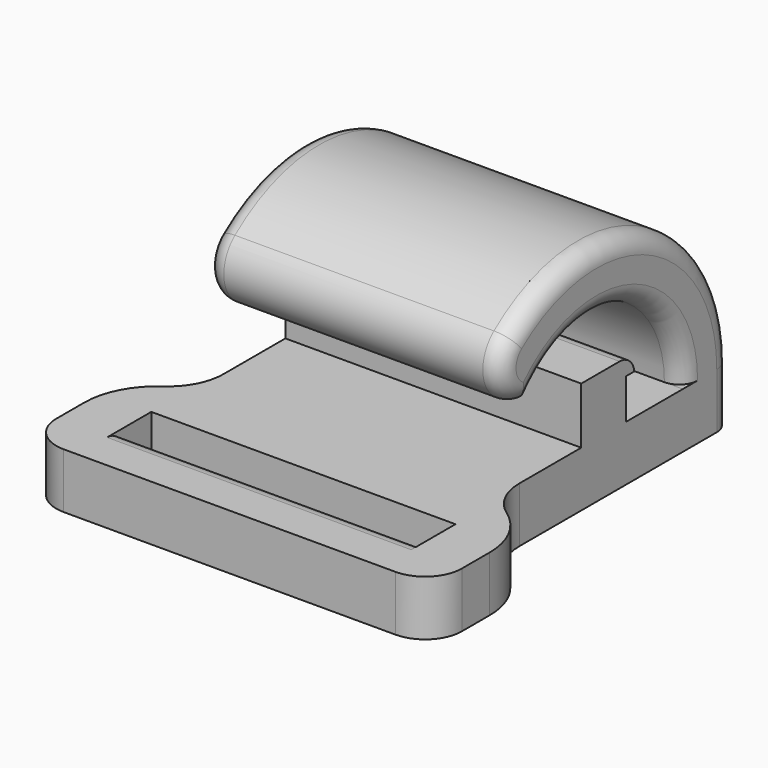
from build123d import *

# Parameters (mm, degrees)
F3_DEPTH       = 16.05
F4_W           = 5.4241176695
F4_H           = 3.5927895224
F5_DEPTH       = 25
F5_DEPTH_BACK  = 25
F6_T1_DEPTH    = 38.39224199
F8_DEPTH       = 8.025
F8_DEPTH_BACK  = 8.025
F9_T1_DEPTH    = 21.0152154422
F11_W          = 7.7522003338
F11_H          = 3
F12_DEPTH      = 11
F12_DEPTH_BACK = 11
F13_W          = 16.5
F13_H          = 2
F14_DEPTH      = 25
F15_R          = 1
F16_T1_DEPTH   = 22.3322108151
F17_T3_ANGLE   = 128.6137584612
F17_T6_ANGLE   = 128.6137584612
F17_T9_ANGLE   = 166.6195765903
F17_T12_ANGLE  = 166.6195765903
F17_T15_ANGLE  = 208.6372867238
F17_T18_ANGLE  = 208.6372867238
F17_T21_DEPTH  = 5.5
F17_T24_DEPTH  = 5.5
F18_R          = 2
F19_R          = 3


# Not quite as in the source:
# - a fillet or chamfer that OpenCascade refuses, or shapes differently, is made with other operations: its cross-section is extruded or revolved along the edge and cut away or added


with BuildPart() as f3:
    # F2 (on line) → F3 (new body)
    with BuildSketch(Plane.YZ.offset(-8.025)):
        with BuildLine():
            Line((30.8775485963, 0), (34.1775485963, 0))
            ThreePointArc((34.1775485963, 0), (25.0275485963, 9.15), (15.8775485963, 0))
            Line((15.8775485963, 0), (19.1775485963, 0))
            ThreePointArc((19.1775485963, 0), (25.0275485963, 5.85), (30.8775485963, 0))
        make_face()
    extrude(amount=F3_DEPTH)

    # F4 (on Right) → F5 (cut, two sides)
    with BuildSketch(Plane.YZ) as f5_sk:
        with Locations((17.9089335725, 1.7963947612)):
            Rectangle(F4_W, F4_H)
    extrude(amount=-F5_DEPTH, mode=Mode.SUBTRACT)
    extrude(f5_sk.sketch, amount=F5_DEPTH_BACK, mode=Mode.SUBTRACT)

    # F6: fillet of radius 2 on 1 edges, made by hand

    # F6_s2 → F6_t1 (cut)
    with BuildSketch(Plane.YZ.offset(-19.196120995)):
        with BuildLine():
            ThreePointArc((19.3173332992, 7.1495413322), (18.6537711345, 4.9990791235), (20.4108004498, 3.5927895224))
            Line((20.4108004498, 3.5927895224), (16.6124215356, 3.5927895224))
            ThreePointArc((16.6124215356, 3.5927895224), (17.7444211746, 5.5388225246), (19.3173332992, 7.1495413322))
        make_face()
    extrude(amount=F6_T1_DEPTH, mode=Mode.SUBTRACT)

    # F7 (on Right) → F8 (join, two sides)
    with BuildSketch(Plane.YZ) as f8_sk:
        Polygon((34.1775485963, 0), (27.0130820572, 0), (23.9856019616, 0), (10.1775485963, 0), (10.1775485963, -3), (34.1775485963, -3), align=None)
        Polygon((23.9856019616, 0), (27.0130820572, 0), (27.0130820572, 2.18), (27.5856019616, 2.18), (27.5856019616, 3.0622484628), (23.9856019616, 3.0622484628), (23.9856019616, 2.18), align=None)
    extrude(amount=F8_DEPTH)
    extrude(f8_sk.sketch, amount=-F8_DEPTH_BACK)

    # F9: fillet of radius 1 on 1 edges, made by hand

    # F9_s2 → F9_t1 (cut)
    with BuildSketch(Plane.YZ.offset(-10.5076077211)):
        with BuildLine():
            ThreePointArc((27.5856019616, 2.18), (27.2567307119, 2.8098284041), (26.5925588732, 3.0622484628))
            Line((26.5925588732, 3.0622484628), (27.5856019616, 3.0622484628))
            Line((27.5856019616, 3.0622484628), (27.5856019616, 2.18))
        make_face()
    extrude(amount=F9_T1_DEPTH, mode=Mode.SUBTRACT)

    # F10: union 

    # F11 (on Right) → F12 (join, two sides)
    with BuildSketch(Plane.YZ) as f12_sk:
        with Locations((14.0536487631, -1.5)):
            Rectangle(F11_W, F11_H)
    extrude(amount=F12_DEPTH)
    extrude(f12_sk.sketch, amount=-F12_DEPTH_BACK)

    # F13 (on Top) → F14 (cut)
    with BuildSketch(Plane.XY):
        with Locations((0, 14.1775485963)):
            Rectangle(F13_W, F13_H)
    extrude(amount=-F14_DEPTH, mode=Mode.SUBTRACT)

    # F15
    f15_edges = [f3.edges().sort_by_distance(p)[0] for p in [
        (0, 13.177549, -3),
        (0, 13.177549, 0),
    ]]
    fillet(f15_edges, radius=F15_R)

    # F16: fillet of radius 4 on 2 edges, made by hand

    # F16_s2 → F16_t1 (cut)
    with BuildSketch(Plane.XY.offset(-12.6661054076)):
        with BuildLine():
            ThreePointArc((-8.025, 17.92974893), (-10.1701734968, 16.5025689505), (-11, 14.063306767))
            Line((-11, 14.063306767), (-11, 17.92974893))
            Line((-11, 17.92974893), (-8.025, 17.92974893))
        make_face()
        with BuildLine():
            ThreePointArc((8.025, 17.92974893), (10.1701734968, 16.5025689505), (11, 14.063306767))
            Line((11, 14.063306767), (11, 17.92974893))
            Line((11, 17.92974893), (8.025, 17.92974893))
        make_face()
    extrude(amount=F16_T1_DEPTH, mode=Mode.SUBTRACT)

    # F17: fillet of radius 1 on 8 edges, made by hand


with BuildPart() as f17_tool1:
    # F17_s2 → F17_t3 (revolve)
    with BuildSketch(Plane.XY):
        with BuildLine():
            ThreePointArc((-7.025, 34.1775485963), (-7.7321067812, 33.8846553774), (-8.025, 33.1775485963))
            Line((-8.025, 33.1775485963), (-8.025, 34.1775485963))
            Line((-8.025, 34.1775485963), (-7.025, 34.1775485963))
        make_face()
    revolve(axis=Axis((-8.025, 25.0275485963, 0), (1, 0, 0)), revolution_arc=F17_T3_ANGLE)


with BuildPart() as f17_tool4:
    # F17_s5 → F17_t6 (revolve)
    with BuildSketch(Plane.XY):
        with BuildLine():
            ThreePointArc((7.025, 34.1775485963), (7.7321067812, 33.8846553774), (8.025, 33.1775485963))
            Line((8.025, 33.1775485963), (8.025, 34.1775485963))
            Line((8.025, 34.1775485963), (7.025, 34.1775485963))
        make_face()
    revolve(axis=Axis((8.025, 25.0275485963, 0), (1, 0, 0)), revolution_arc=F17_T6_ANGLE)


with BuildPart() as f17_tool7:
    # F17_s8 → F17_t9 (revolve)
    with BuildSketch(Plane(origin=(0, 1.3403038382, 5.634545684), x_dir=(1, 0, 0), z_dir=(0, -0.2314155158, -0.9728550041))):
        with BuildLine():
            ThreePointArc((-7.025, -18.4981758925), (-7.7321067812, -18.2052826737), (-8.025, -17.4981758925))
            Line((-8.025, -17.4981758925), (-8.025, -18.4981758925))
            Line((-8.025, -18.4981758925), (-7.025, -18.4981758925))
        make_face()
    revolve(axis=Axis((-8.025, 25.0275485963, 0), (-1, 0, 0)), revolution_arc=F17_T9_ANGLE)


with BuildPart() as f17_tool10:
    # F17_s11 → F17_t12 (revolve)
    with BuildSketch(Plane(origin=(0, 1.3403038382, 5.634545684), x_dir=(1, 0, 0), z_dir=(0, -0.2314155158, -0.9728550041))):
        with BuildLine():
            ThreePointArc((7.025, -18.4981758925), (7.7321067812, -18.2052826737), (8.025, -17.4981758925))
            Line((8.025, -17.4981758925), (8.025, -18.4981758925))
            Line((8.025, -18.4981758925), (7.025, -18.4981758925))
        make_face()
    revolve(axis=Axis((8.025, 25.0275485963, 0), (-1, 0, 0)), revolution_arc=F17_T12_ANGLE)


with BuildPart() as f17_tool13:
    # F17_s14 → F17_t15 (revolve)
    with BuildSketch(Plane(origin=(0, 5.0675252641, 12.0852942927), x_dir=(1, 0, 0), z_dir=(0, 0.3866941389, 0.9222080259))):
        with BuildLine():
            ThreePointArc((-7.025, 18.8052566142), (-7.7321067812, 18.5123633954), (-8.025, 17.8052566142))
            Line((-8.025, 17.8052566142), (-8.025, 18.8052566142))
            Line((-8.025, 18.8052566142), (-7.025, 18.8052566142))
        make_face()
    revolve(axis=Axis((-8.025, 20.5654677903, 5.5868000574), (-1, 0, 0)), revolution_arc=F17_T15_ANGLE)


with BuildPart() as f17_tool16:
    # F17_s17 → F17_t18 (revolve)
    with BuildSketch(Plane(origin=(0, 5.0675252641, 12.0852942927), x_dir=(1, 0, 0), z_dir=(0, 0.3866941389, 0.9222080259))):
        with BuildLine():
            ThreePointArc((7.025, 18.8052566142), (7.7321067812, 18.5123633954), (8.025, 17.8052566142))
            Line((8.025, 17.8052566142), (8.025, 18.8052566142))
            Line((8.025, 18.8052566142), (7.025, 18.8052566142))
        make_face()
    revolve(axis=Axis((8.025, 20.5654677903, 5.5868000574), (-1, 0, 0)), revolution_arc=F17_T18_ANGLE)


with BuildPart() as f17_tool19:
    # F17_s20 → F17_t21 (new body)
    with BuildSketch(Plane.XY.offset(-5.5)):
        with BuildLine():
            ThreePointArc((7.025, 34.1775485963), (7.7321067812, 33.8846553774), (8.025, 33.1775485963))
            Line((8.025, 33.1775485963), (8.025, 34.1775485963))
            Line((8.025, 34.1775485963), (7.025, 34.1775485963))
        make_face()
    extrude(amount=F17_T21_DEPTH)


with BuildPart() as f17_tool22:
    # F17_s23 → F17_t24 (new body)
    with BuildSketch(Plane.XY.offset(-5.5)):
        with BuildLine():
            ThreePointArc((-7.025, 34.1775485963), (-7.7321067812, 33.8846553774), (-8.025, 33.1775485963))
            Line((-8.025, 33.1775485963), (-8.025, 34.1775485963))
            Line((-8.025, 34.1775485963), (-7.025, 34.1775485963))
        make_face()
    extrude(amount=F17_T24_DEPTH)


with BuildPart() as f3_1:
    add(f3.part)

    # F17_t25: cut F17_tool1, F17_tool4, F17_tool7, F17_tool10, F17_tool13, F17_tool16, F17_tool19, F17_tool22
    add([f17_tool1.part, f17_tool4.part, f17_tool7.part, f17_tool10.part, f17_tool13.part, f17_tool16.part, f17_tool19.part, f17_tool22.part], mode=Mode.SUBTRACT)

    # F18
    f18_edges = [f3_1.edges().sort_by_distance(p)[0] for p in [
        (-11, 10.177549, -1.5),
        (11, 10.177549, -1.5),
    ]]
    fillet(f18_edges, radius=F18_R)

    # F19
    f19_edges = [f3_1.edges().sort_by_distance(p)[0] for p in [
        (-8.025, 17.929749, -1.5),
        (8.025, 17.929749, -1.5),
    ]]
    fillet(f19_edges, radius=F19_R)


solid = f3_1.part
